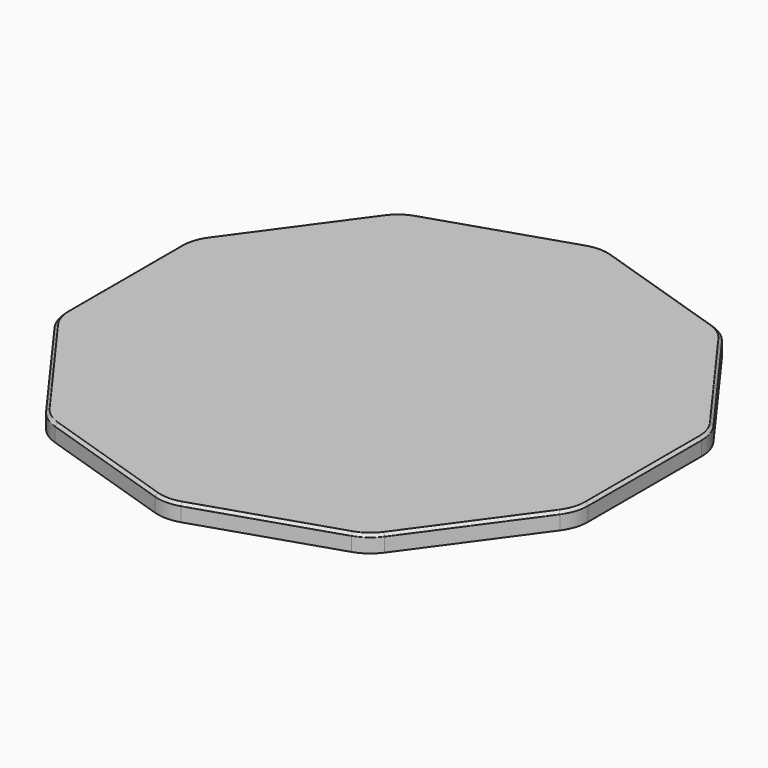
from build123d import *

# Parameters (mm, degrees)
F1_DEPTH       = 5.08
F2_R           = 6.35
F3_R           = 1.27
F5_DEPTH       = 1.27
F7_D           = 3.81
F7_DEPTH       = 12.7
F7_CBORE_D     = 5.08
F7_CBORE_DEPTH = 1.27
F7_TIP         = 1.1446394792
F8_DEPTH       = 25.4
F9_DEPTH       = 6.35
F10_DEPTH      = 1.016
F11_T1_DEPTH   = 12.8274282372
F11_T3_DEPTH   = 12.8274282372
F11_T5_DEPTH   = 12.8274282372
F11_T7_DEPTH   = 12.8274282372
F11_T9_DEPTH   = 12.8274282372
F11_T11_DEPTH  = 12.8274282372
F11_T13_DEPTH  = 12.8274282372
F11_T15_DEPTH  = 12.8274282372
F11_T17_DEPTH  = 12.8274282372
F11_T20_ANGLE  = 36
F11_T22_ANGLE  = 36
F11_T24_ANGLE  = 36
F11_T26_ANGLE  = 36
F11_T28_ANGLE  = 36
F11_T30_ANGLE  = 36
F11_T32_ANGLE  = 36
F11_T34_ANGLE  = 36
F11_T36_ANGLE  = 36
F11_T38_ANGLE  = 36


# Not quite as in the source:
# - a fillet or chamfer that OpenCascade refuses, or shapes differently, is made with other operations: its cross-section is extruded or revolved along the edge and cut away or added


with BuildPart() as f1:
    # F0 (on Top) → F1 (new body, symmetric)
    with BuildSketch(Plane.XY):
        Polygon((26.089382355, -8.4769541897), (26.089382355, 8.4769541897), (16.1241250409, 22.1929541897), (0, 27.432), (-16.1241250409, 22.1929541897), (-26.089382355, 8.4769541897), (-26.089382355, -8.4769541897), (-16.1241250409, -22.1929541897), (0, -27.432), (16.1241250409, -22.1929541897), align=None)
    extrude(amount=F1_DEPTH, both=True)

    # F2
    f2_edges = [f1.edges().sort_by_distance(p)[0] for p in [
        (-16.124125, -22.192954, 0),
        (-26.089382, -8.476954, 0),
        (-26.089382, 8.476954, 0),
        (-16.124125, 22.192954, 0),
        (0, 27.432, 0),
        (16.124125, 22.192954, 0),
        (26.089382, 8.476954, 0),
        (16.124125, -22.192954, 0),
        (0, -27.432, 0),
        (26.089382, -8.476954, 0),
    ]]
    fillet(f2_edges, radius=F2_R)

    # F3
    f3_edges = [f1.edges().sort_by_distance(p)[0] for p in [
        (21.106754, -15.334954, -5.08),
        (15.932046, -21.928579, -5.08),
        (25.778591, -8.375972, -5.08),
        (8.062063, -24.812477, -5.08),
        (26.089382, 0, -5.08),
        (0, -27.105215, -5.08),
        (25.778591, 8.375972, -5.08),
        (-8.062063, -24.812477, -5.08),
        (21.106754, 15.334954, -5.08),
        (-15.932046, -21.928579, -5.08),
        (15.932046, 21.928579, -5.08),
        (-21.106754, -15.334954, -5.08),
        (8.062063, 24.812477, -5.08),
        (-25.778591, -8.375972, -5.08),
        (0, 27.105215, -5.08),
        (-26.089382, 0, -5.08),
        (-8.062063, 24.812477, -5.08),
        (-25.778591, 8.375972, -5.08),
        (-15.932046, 21.928579, -5.08),
        (-21.106754, 15.334954, -5.08),
    ]]
    fillet(f3_edges, radius=F3_R)

    # F4 (on face) → F5 (cut)
    with BuildSketch(Plane.XY.offset(5.08)):
        with BuildLine():
            ThreePointArc((-23.549382355, -6.4137141186), (-23.3629076821, -7.5910688672), (-22.8217371036, -8.6531759298))
            Line((-22.8217371036, -8.6531759298), (-15.2819639609, -19.0307833679))
            ThreePointArc((-15.2819639609, -19.0307833679), (-14.4390710236, -19.8736763052), (-13.3769639609, -20.4148468837))
            Line((-13.3769639609, -20.4148468837), (-1.1773547486, -24.3787402032))
            ThreePointArc((-1.1773547486, -24.3787402032), (0, -24.5652148761), (1.1773547486, -24.3787402032))
            Line((1.1773547486, -24.3787402032), (13.3769639609, -20.4148468837))
            ThreePointArc((13.3769639609, -20.4148468837), (14.4390710236, -19.8736763052), (15.2819639609, -19.0307833679))
            Line((15.2819639609, -19.0307833679), (22.8217371036, -8.6531759298))
            ThreePointArc((22.8217371036, -8.6531759298), (23.3629076821, -7.5910688672), (23.549382355, -6.4137141186))
            Line((23.549382355, -6.4137141186), (23.549382355, 6.4137141186))
            ThreePointArc((23.549382355, 6.4137141186), (23.3629076821, 7.5910688672), (22.8217371036, 8.6531759298))
            Line((22.8217371036, 8.6531759298), (15.2819639609, 19.0307833679))
            ThreePointArc((15.2819639609, 19.0307833679), (14.4390710236, 19.8736763052), (13.3769639609, 20.4148468837))
            Line((13.3769639609, 20.4148468837), (1.1773547486, 24.3787402032))
            ThreePointArc((1.1773547486, 24.3787402032), (0, 24.5652148761), (-1.1773547486, 24.3787402032))
            Line((-1.1773547486, 24.3787402032), (-13.3769639609, 20.4148468837))
            ThreePointArc((-13.3769639609, 20.4148468837), (-14.4390710236, 19.8736763052), (-15.2819639609, 19.0307833679))
            Line((-15.2819639609, 19.0307833679), (-22.8217371036, 8.6531759298))
            ThreePointArc((-22.8217371036, 8.6531759298), (-23.3629076821, 7.5910688672), (-23.549382355, 6.4137141186))
            Line((-23.549382355, 6.4137141186), (-23.549382355, -6.4137141186))
        make_face()
    extrude(amount=-F5_DEPTH, mode=Mode.SUBTRACT)

    # F7
    with Locations(Plane.YZ.offset(26.089382355)):
        with Locations((0, 0)):
            CounterBoreHole(F7_D / 2, F7_CBORE_D / 2, F7_CBORE_DEPTH, depth=F7_DEPTH)
            with Locations((0, 0, -(F7_DEPTH + F7_TIP / 2))):  # 118° drill point
                Cone(0, F7_D / 2, F7_TIP, mode=Mode.SUBTRACT)

    # F8 (cut): a face of the model
    f8_faces = [f1.faces().sort_by_distance(p)[0] for p in [
        (20.4980312163, -14.892691419, 5.08),
    ]]
    extrude(f8_faces, amount=-F8_DEPTH, mode=Mode.SUBTRACT)

    # F9 (cut): a face of the model
    f9_faces = [f1.faces().sort_by_distance(p)[0] for p in [
        (0, 0, 3.81),
    ]]
    extrude(f9_faces, amount=-F9_DEPTH, mode=Mode.SUBTRACT)

    # F10 (cut): a face of the model
    f10_faces = [f1.faces().sort_by_distance(p)[0] for p in [
        (0, 0, -2.54),
    ]]
    extrude(f10_faces, amount=-F10_DEPTH, mode=Mode.SUBTRACT)

    # F11: fillet of radius 0.254 on 20 edges, made by hand

    # F11_s2 → F11_t1 (cut)
    with BuildSketch(Plane(origin=(3.7698865713, 5.188803719, 0), x_dir=(0, 0, 1), z_dir=(-0.5877852523, -0.8090169944, 0))):
        with BuildLine():
            add(Edge.make_bspline(
                [(-3.81, 23.549382355), (-3.556, 23.549382355), (-3.556, 23.295382355)],
                knots=[0, 0, 0, 1, 1, 1], degree=2, weights=[1, 0.1111111111, 1]))
            Line((-3.556, 23.295382355), (-3.556, 23.549382355))
            Line((-3.556, 23.549382355), (-3.81, 23.549382355))
        make_face()
    extrude(amount=F11_T1_DEPTH, mode=Mode.SUBTRACT)

    # F11_s4 → F11_t3 (cut)
    with BuildSketch(Plane.XZ.offset(-6.4137141186)):
        with BuildLine():
            add(Edge.make_bspline(
                [(-23.549382355, -3.81), (-23.549382355, -3.556), (-23.295382355, -3.556)],
                knots=[0, 0, 0, 1, 1, 1], degree=2, weights=[1, 0.1111111111, 1]))
            Line((-23.295382355, -3.556), (-23.549382355, -3.556))
            Line((-23.549382355, -3.556), (-23.549382355, -3.81))
        make_face()
        with BuildLine():
            add(Edge.make_bspline(
                [(23.549382355, -3.81), (23.549382355, -3.556), (23.295382355, -3.556)],
                knots=[0, 0, 0, 1, 1, 1], degree=2, weights=[1, 0.1111111111, 1]))
            Line((23.295382355, -3.556), (23.549382355, -3.556))
            Line((23.549382355, -3.556), (23.549382355, -3.81))
        make_face()
    extrude(amount=F11_T3_DEPTH, mode=Mode.SUBTRACT)

    # F11_s6 → F11_t5 (cut)
    with BuildSketch(Plane(origin=(-3.7698865713, 5.188803719, 0), x_dir=(0, 0, 1), z_dir=(0.5877852523, -0.8090169944, 0))):
        with BuildLine():
            add(Edge.make_bspline(
                [(-3.81, 23.549382355), (-3.556, 23.549382355), (-3.556, 23.295382355)],
                knots=[0, 0, 0, 1, 1, 1], degree=2, weights=[1, 0.1111111111, 1]))
            Line((-3.556, 23.295382355), (-3.556, 23.549382355))
            Line((-3.556, 23.549382355), (-3.81, 23.549382355))
        make_face()
    extrude(amount=F11_T5_DEPTH, mode=Mode.SUBTRACT)

    # F11_s8 → F11_t7 (cut)
    with BuildSketch(Plane(origin=(-6.0998046062, 1.9819466597, 0), x_dir=(0, 0, 1), z_dir=(0.9510565163, -0.3090169944, 0))):
        with BuildLine():
            add(Edge.make_bspline(
                [(-3.81, 23.549382355), (-3.556, 23.549382355), (-3.556, 23.295382355)],
                knots=[0, 0, 0, 1, 1, 1], degree=2, weights=[1, 0.1111111111, 1]))
            Line((-3.556, 23.295382355), (-3.556, 23.549382355))
            Line((-3.556, 23.549382355), (-3.81, 23.549382355))
        make_face()
    extrude(amount=F11_T7_DEPTH, mode=Mode.SUBTRACT)

    # F11_s10 → F11_t9 (cut)
    with BuildSketch(Plane(origin=(-6.0998046062, -1.9819466597, 0), x_dir=(0, 0, 1), z_dir=(0.9510565163, 0.3090169944, 0))):
        with BuildLine():
            add(Edge.make_bspline(
                [(-3.81, 23.549382355), (-3.556, 23.549382355), (-3.556, 23.295382355)],
                knots=[0, 0, 0, 1, 1, 1], degree=2, weights=[1, 0.1111111111, 1]))
            Line((-3.556, 23.295382355), (-3.556, 23.549382355))
            Line((-3.556, 23.549382355), (-3.81, 23.549382355))
        make_face()
    extrude(amount=F11_T9_DEPTH, mode=Mode.SUBTRACT)

    # F11_s12 → F11_t11 (cut)
    with BuildSketch(Plane(origin=(-3.7698865713, -5.188803719, 0), x_dir=(0, 0, 1), z_dir=(0.5877852523, 0.8090169944, 0))):
        with BuildLine():
            add(Edge.make_bspline(
                [(-3.81, 23.549382355), (-3.556, 23.549382355), (-3.556, 23.295382355)],
                knots=[0, 0, 0, 1, 1, 1], degree=2, weights=[1, 0.1111111111, 1]))
            Line((-3.556, 23.295382355), (-3.556, 23.549382355))
            Line((-3.556, 23.549382355), (-3.81, 23.549382355))
        make_face()
    extrude(amount=F11_T11_DEPTH, mode=Mode.SUBTRACT)

    # F11_s14 → F11_t13 (cut)
    with BuildSketch(Plane(origin=(3.7698865713, -5.188803719, 0), x_dir=(0, 0, 1), z_dir=(-0.5877852523, 0.8090169944, 0))):
        with BuildLine():
            add(Edge.make_bspline(
                [(-3.81, 23.549382355), (-3.556, 23.549382355), (-3.556, 23.295382355)],
                knots=[0, 0, 0, 1, 1, 1], degree=2, weights=[1, 0.1111111111, 1]))
            Line((-3.556, 23.295382355), (-3.556, 23.549382355))
            Line((-3.556, 23.549382355), (-3.81, 23.549382355))
        make_face()
    extrude(amount=F11_T13_DEPTH, mode=Mode.SUBTRACT)

    # F11_s16 → F11_t15 (cut)
    with BuildSketch(Plane(origin=(6.0998046062, -1.9819466597, 0), x_dir=(0, 0, 1), z_dir=(-0.9510565163, 0.3090169944, 0))):
        with BuildLine():
            add(Edge.make_bspline(
                [(-3.81, 23.549382355), (-3.556, 23.549382355), (-3.556, 23.295382355)],
                knots=[0, 0, 0, 1, 1, 1], degree=2, weights=[1, 0.1111111111, 1]))
            Line((-3.556, 23.295382355), (-3.556, 23.549382355))
            Line((-3.556, 23.549382355), (-3.81, 23.549382355))
        make_face()
    extrude(amount=F11_T15_DEPTH, mode=Mode.SUBTRACT)

    # F11_s18 → F11_t17 (cut)
    with BuildSketch(Plane(origin=(6.0998046062, 1.9819466597, 0), x_dir=(0, 0, 1), z_dir=(-0.9510565163, -0.3090169944, 0))):
        with BuildLine():
            add(Edge.make_bspline(
                [(-3.81, 23.549382355), (-3.556, 23.549382355), (-3.556, 23.295382355)],
                knots=[0, 0, 0, 1, 1, 1], degree=2, weights=[1, 0.1111111111, 1]))
            Line((-3.556, 23.295382355), (-3.556, 23.549382355))
            Line((-3.556, 23.549382355), (-3.81, 23.549382355))
        make_face()
    extrude(amount=F11_T17_DEPTH, mode=Mode.SUBTRACT)

    # F11_s19 → F11_t20 (revolve, cut)
    with BuildSketch(Plane(origin=(-6.0998046062, -1.9819466597, 0), x_dir=(0, 0, 1), z_dir=(0.9510565163, 0.3090169944, 0))):
        with BuildLine():
            add(Edge.make_bspline(
                [(-3.81, -23.549382355), (-3.556, -23.549382355), (-3.556, -23.295382355)],
                knots=[0, 0, 0, 1, 1, 1], degree=2, weights=[1, 0.1111111111, 1]))
            Line((-3.556, -23.295382355), (-3.556, -23.549382355))
            Line((-3.556, -23.549382355), (-3.81, -23.549382355))
        make_face()
    revolve(axis=Axis((-12.1996092123, 16.7913215567, -3.556), (0, 0, 1)), revolution_arc=F11_T20_ANGLE, mode=Mode.SUBTRACT)

    # F11_s21 → F11_t22 (revolve, cut)
    with BuildSketch(Plane(origin=(-3.7698865713, -5.188803719, 0), x_dir=(0, 0, 1), z_dir=(0.5877852523, 0.8090169944, 0))):
        with BuildLine():
            add(Edge.make_bspline(
                [(-3.81, -23.549382355), (-3.556, -23.549382355), (-3.556, -23.295382355)],
                knots=[0, 0, 0, 1, 1, 1], degree=2, weights=[1, 0.1111111111, 1]))
            Line((-3.556, -23.295382355), (-3.556, -23.549382355))
            Line((-3.556, -23.549382355), (-3.81, -23.549382355))
        make_face()
    revolve(axis=Axis((-19.739382355, 6.4137141186, -3.556), (0, 0, 1)), revolution_arc=F11_T22_ANGLE, mode=Mode.SUBTRACT)

    # F11_s23 → F11_t24 (revolve, cut)
    with BuildSketch(Plane.XZ.offset(6.4137141186)):
        with BuildLine():
            add(Edge.make_bspline(
                [(-23.549382355, -3.81), (-23.549382355, -3.556), (-23.295382355, -3.556)],
                knots=[0, 0, 0, 1, 1, 1], degree=2, weights=[1, 0.1111111111, 1]))
            Line((-23.295382355, -3.556), (-23.549382355, -3.556))
            Line((-23.549382355, -3.556), (-23.549382355, -3.81))
        make_face()
    revolve(axis=Axis((-19.739382355, -6.4137141186, -3.556), (0, 0, 1)), revolution_arc=F11_T24_ANGLE, mode=Mode.SUBTRACT)

    # F11_s25 → F11_t26 (revolve, cut)
    with BuildSketch(Plane(origin=(3.7698865713, -5.188803719, 0), x_dir=(0, 0, 1), z_dir=(-0.5877852523, 0.8090169944, 0))):
        with BuildLine():
            add(Edge.make_bspline(
                [(-3.81, -23.549382355), (-3.556, -23.549382355), (-3.556, -23.295382355)],
                knots=[0, 0, 0, 1, 1, 1], degree=2, weights=[1, 0.1111111111, 1]))
            Line((-3.556, -23.295382355), (-3.556, -23.549382355))
            Line((-3.556, -23.549382355), (-3.81, -23.549382355))
        make_face()
    revolve(axis=Axis((-12.1996092123, -16.7913215567, -3.556), (0, 0, 1)), revolution_arc=F11_T26_ANGLE, mode=Mode.SUBTRACT)

    # F11_s27 → F11_t28 (revolve, cut)
    with BuildSketch(Plane(origin=(6.0998046062, -1.9819466597, 0), x_dir=(0, 0, 1), z_dir=(-0.9510565163, 0.3090169944, 0))):
        with BuildLine():
            add(Edge.make_bspline(
                [(-3.81, -23.549382355), (-3.556, -23.549382355), (-3.556, -23.295382355)],
                knots=[0, 0, 0, 1, 1, 1], degree=2, weights=[1, 0.1111111111, 1]))
            Line((-3.556, -23.295382355), (-3.556, -23.549382355))
            Line((-3.556, -23.549382355), (-3.81, -23.549382355))
        make_face()
    revolve(axis=Axis((0, -20.7552148761, -3.556), (0, 0, 1)), revolution_arc=F11_T28_ANGLE, mode=Mode.SUBTRACT)

    # F11_s29 → F11_t30 (revolve, cut)
    with BuildSketch(Plane(origin=(6.0998046062, 1.9819466597, 0), x_dir=(0, 0, 1), z_dir=(-0.9510565163, -0.3090169944, 0))):
        with BuildLine():
            add(Edge.make_bspline(
                [(-3.81, -23.549382355), (-3.556, -23.549382355), (-3.556, -23.295382355)],
                knots=[0, 0, 0, 1, 1, 1], degree=2, weights=[1, 0.1111111111, 1]))
            Line((-3.556, -23.295382355), (-3.556, -23.549382355))
            Line((-3.556, -23.549382355), (-3.81, -23.549382355))
        make_face()
    revolve(axis=Axis((12.1996092123, -16.7913215567, -3.556), (0, 0, 1)), revolution_arc=F11_T30_ANGLE, mode=Mode.SUBTRACT)

    # F11_s31 → F11_t32 (revolve, cut)
    with BuildSketch(Plane(origin=(3.7698865713, 5.188803719, 0), x_dir=(0, 0, 1), z_dir=(-0.5877852523, -0.8090169944, 0))):
        with BuildLine():
            add(Edge.make_bspline(
                [(-3.81, -23.549382355), (-3.556, -23.549382355), (-3.556, -23.295382355)],
                knots=[0, 0, 0, 1, 1, 1], degree=2, weights=[1, 0.1111111111, 1]))
            Line((-3.556, -23.295382355), (-3.556, -23.549382355))
            Line((-3.556, -23.549382355), (-3.81, -23.549382355))
        make_face()
    revolve(axis=Axis((19.739382355, -6.4137141186, -3.556), (0, 0, 1)), revolution_arc=F11_T32_ANGLE, mode=Mode.SUBTRACT)

    # F11_s33 → F11_t34 (revolve, cut)
    with BuildSketch(Plane.XZ.offset(-6.4137141186)):
        with BuildLine():
            add(Edge.make_bspline(
                [(23.549382355, -3.81), (23.549382355, -3.556), (23.295382355, -3.556)],
                knots=[0, 0, 0, 1, 1, 1], degree=2, weights=[1, 0.1111111111, 1]))
            Line((23.295382355, -3.556), (23.549382355, -3.556))
            Line((23.549382355, -3.556), (23.549382355, -3.81))
        make_face()
    revolve(axis=Axis((19.739382355, 6.4137141186, -3.556), (0, 0, 1)), revolution_arc=F11_T34_ANGLE, mode=Mode.SUBTRACT)

    # F11_s35 → F11_t36 (revolve, cut)
    with BuildSketch(Plane(origin=(-3.7698865713, 5.188803719, 0), x_dir=(0, 0, 1), z_dir=(0.5877852523, -0.8090169944, 0))):
        with BuildLine():
            add(Edge.make_bspline(
                [(-3.81, -23.549382355), (-3.556, -23.549382355), (-3.556, -23.295382355)],
                knots=[0, 0, 0, 1, 1, 1], degree=2, weights=[1, 0.1111111111, 1]))
            Line((-3.556, -23.295382355), (-3.556, -23.549382355))
            Line((-3.556, -23.549382355), (-3.81, -23.549382355))
        make_face()
    revolve(axis=Axis((12.1996092123, 16.7913215567, -3.556), (0, 0, 1)), revolution_arc=F11_T36_ANGLE, mode=Mode.SUBTRACT)

    # F11_s37 → F11_t38 (revolve, cut)
    with BuildSketch(Plane(origin=(-6.0998046062, 1.9819466597, 0), x_dir=(0, 0, 1), z_dir=(0.9510565163, -0.3090169944, 0))):
        with BuildLine():
            add(Edge.make_bspline(
                [(-3.81, -23.549382355), (-3.556, -23.549382355), (-3.556, -23.295382355)],
                knots=[0, 0, 0, 1, 1, 1], degree=2, weights=[1, 0.1111111111, 1]))
            Line((-3.556, -23.295382355), (-3.556, -23.549382355))
            Line((-3.556, -23.549382355), (-3.81, -23.549382355))
        make_face()
    revolve(axis=Axis((0, 20.7552148761, -3.556), (0, 0, 1)), revolution_arc=F11_T38_ANGLE, mode=Mode.SUBTRACT)


solid = f1.part
